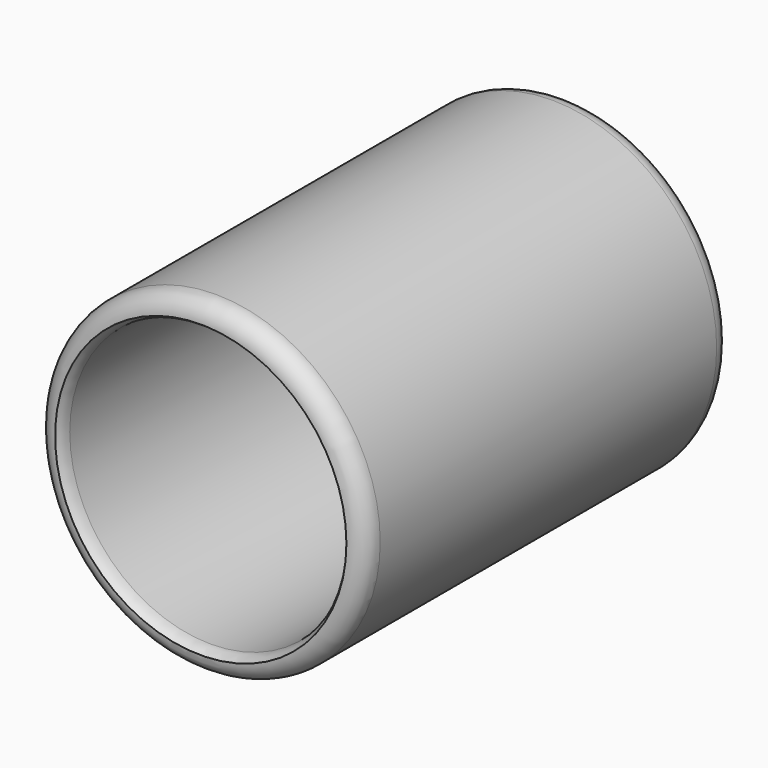
from build123d import *

# Parameters (mm, degrees)
F0_R     = 44.45
F0_R_2   = 38.1
F1_DEPTH = 123.825
F2_R     = 44.45
F3_DEPTH = 6.35
F4_R     = 5.08


# Not quite as in the source:
# - a fillet or chamfer that OpenCascade refuses, or shapes differently, is made with other operations: its cross-section is extruded or revolved along the edge and cut away or added


with BuildPart() as f1:
    # F0 (on Front) → F1 (new body)
    with BuildSketch(Plane.XZ):
        Circle(F0_R)
        Circle(F0_R_2, mode=Mode.SUBTRACT)
    extrude(amount=F1_DEPTH)

    # F2 (on Front) → F3 (join)
    with BuildSketch(Plane.XZ):
        Circle(F2_R)
    extrude(amount=F3_DEPTH)

    # F4
    f4_edges = [f1.edges().sort_by_distance(p)[0] for p in [
        (-44.45, 0, 0),
        (44.45, -61.9125, 0),
        (-44.45, -123.825, 0),
    ]]
    fillet(f4_edges, radius=F4_R)

    # F5: fillet of radius 5.08 on 2 edges, made by hand

    # F5_s1 → F5_t2 (revolve, cut)
    with BuildSketch(Plane.XY):
        with BuildLine():
            ThreePointArc((39.37, -123.825), (38.4280951188, -122.2609470592), (38.1, -120.4648958349))
            Line((38.1, -120.4648958349), (38.1, -123.825))
            Line((38.1, -123.825), (39.37, -123.825))
        make_face()
    revolve(axis=Axis((0, -123.825, 0), (0, -1, 0)), mode=Mode.SUBTRACT)


solid = f1.part
